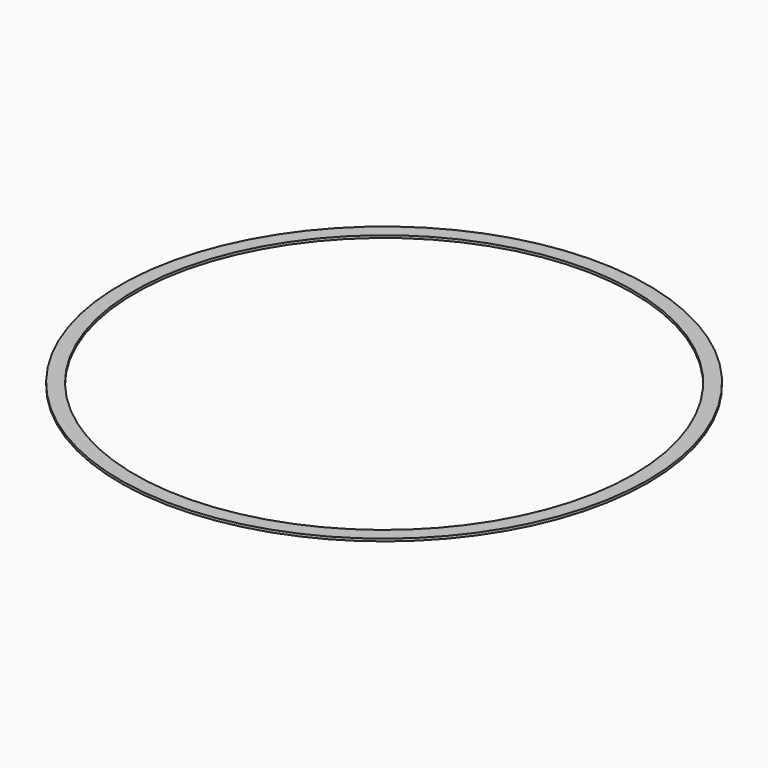
from build123d import *

# Parameters (mm, degrees)
F0_R     = 454.60539
F0_R_2   = 429.20539
F1_DEPTH = 4.2333333333


# Not quite as in the source:
# - a length typed as a fraction of an inch, garbled in the dataset ("3 / 203.2 mm" for 3/8 in), is restored


with BuildPart() as f1:
    # F0 (on Top) → F1 (new body)
    with BuildSketch(Plane.XY):
        Circle(F0_R)
        Circle(F0_R_2, mode=Mode.SUBTRACT)
    extrude(amount=F1_DEPTH)


solid = f1.part
